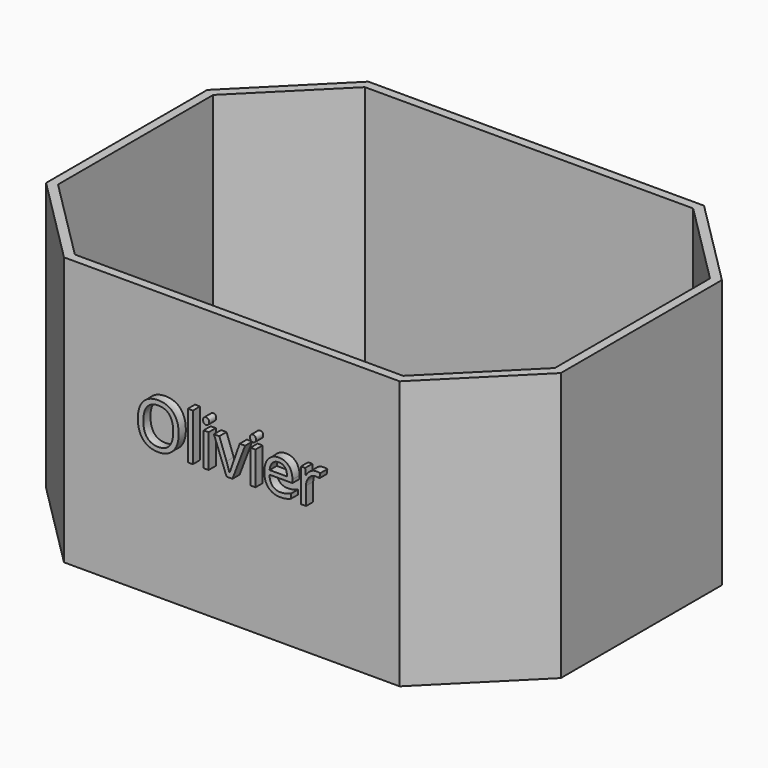
from build123d import *

# Parameters (mm, degrees)
F1_DEPTH     = 76.2
F2_T         = -2.54
F3_TEXT_SIZE = 17.6388888889
F4_DEPTH     = 2.54


# Not quite as in the source:
# - Text() gives the source's letters only with a copy of the font that has no kerning and outlines rounded to 1/6400 em; it was checked with that copy


with BuildPart() as f1:
    # F0 (on Top) → F1 (new body)
    with BuildSketch(Plane.XY):
        Polygon((-47.625, -53.975), (47.625, -53.975), (73.025, -28.575), (73.025, 28.575), (47.625, 53.975), (-47.625, 53.975), (-73.025, 28.575), (-73.025, -28.575), align=None)
    extrude(amount=F1_DEPTH)

    # F2
    f2_openings = [f1.faces().sort_by_distance(p)[0] for p in [
        (0, 0, 76.2),
    ]]
    offset(amount=F2_T, openings=f2_openings)

    # F3 (on face) → F4 (join)
    with BuildSketch(Plane.XZ.offset(53.975)):
        with Locations((-25.7050976562, 38.1)):
            Text('Olivier', F3_TEXT_SIZE, font='Open Sans', text_align=(TextAlign.LEFT, TextAlign.BOTTOM))
    extrude(amount=F4_DEPTH)


solid = f1.part
